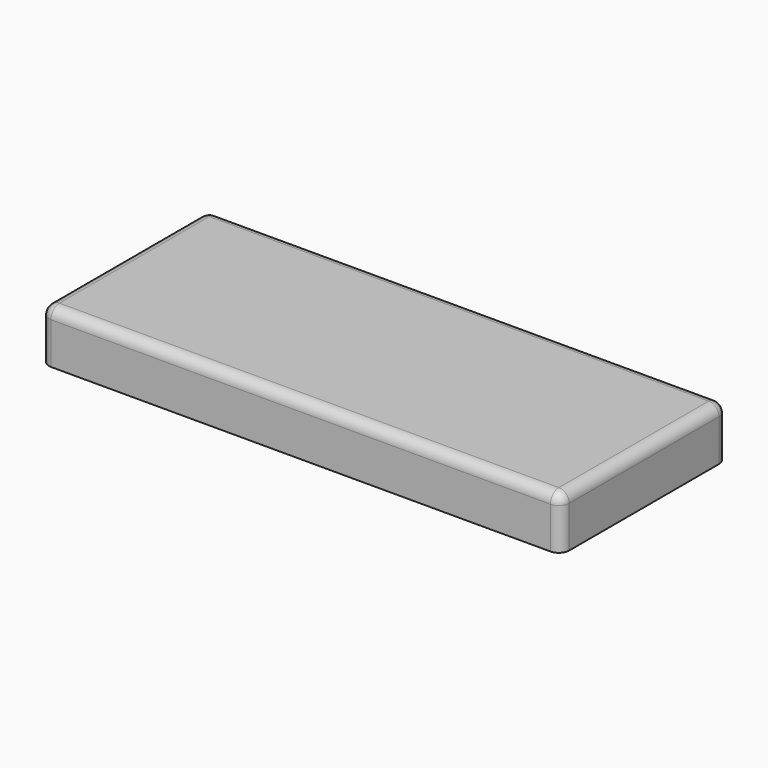
from build123d import *

# Parameters (mm, degrees)
F0_W        = 254
F0_H        = 101.6
F1_DEPTH    = 25.4
F2_R        = 5.08
F3_R        = 5.08
F4_T1_DEPTH = 33.02
F4_S5_W     = 5.08
F4_S5_H     = 5.08
F4_T6_DEPTH = 5.08
F5_T1_DEPTH = 33.02
F5_S5_W     = 5.08
F5_S5_H     = 5.08
F5_T6_DEPTH = 5.08


# Not quite as in the source:
# - a fillet or chamfer that OpenCascade refuses, or shapes differently, is made with other operations: its cross-section is extruded or revolved along the edge and cut away or added


with BuildPart() as f1:
    # F0 (on Top) → F1 (new body)
    with BuildSketch(Plane.XY):
        Rectangle(F0_W, F0_H)
    extrude(amount=F1_DEPTH)

    # F2
    f2_edges = [f1.edges().sort_by_distance(p)[0] for p in [
        (0, -50.8, 25.4),
    ]]
    fillet(f2_edges, radius=F2_R)

    # F3
    f3_edges = [f1.edges().sort_by_distance(p)[0] for p in [
        (127, 2.54, 25.4),
        (0, 50.8, 25.4),
        (-127, 2.54, 25.4),
    ]]
    fillet(f3_edges, radius=F3_R)

    # F4: fillet of radius 5.08 on 1 edges, made by hand

    # F4_s2 → F4_t1 (cut)
    with BuildSketch(Plane.XY.offset(-12.7)):
        with BuildLine():
            ThreePointArc((121.92, 50.8), (125.5121024484, 49.3121024484), (127, 45.72))
            Line((127, 45.72), (127, 50.8))
            Line((127, 50.8), (121.92, 50.8))
        make_face()
    extrude(amount=F4_T1_DEPTH, mode=Mode.SUBTRACT)


with BuildPart() as f4_tool4:
    # F4_s5 → F4_t6 (new body)
    with BuildSketch(Plane.XZ.offset(-45.72)):
        with Locations((124.46, 22.86)):
            Rectangle(F4_S5_W, F4_S5_H)
    extrude(amount=-F4_T6_DEPTH)

    # F4_s7 → F4_t8 (revolve, cut)
    with BuildSketch(Plane(origin=(121.92, 45.72, 20.32), x_dir=(-0.7071067812, 0, -0.7071067812), z_dir=(0.7071067812, 0, -0.7071067812))):
        with BuildLine():
            ThreePointArc((0, -5.08), (5.08, 0), (0, 5.08))
            Line((0, 5.08), (0, -5.08))
        make_face()
    revolve(axis=Axis((121.92, 45.72, 20.32), (0, 1, 0)), mode=Mode.SUBTRACT)


with BuildPart() as f1_1:
    add(f1.part)

    # F4_t3: cut F4_tool4
    add(f4_tool4.part, mode=Mode.SUBTRACT)

    # F5: fillet of radius 5.08 on 1 edges, made by hand

    # F5_s2 → F5_t1 (cut)
    with BuildSketch(Plane.XY.offset(-12.7)):
        with BuildLine():
            ThreePointArc((-127, 45.72), (-125.5121024484, 49.3121024484), (-121.92, 50.8))
            Line((-121.92, 50.8), (-127, 50.8))
            Line((-127, 50.8), (-127, 45.72))
        make_face()
    extrude(amount=F5_T1_DEPTH, mode=Mode.SUBTRACT)


with BuildPart() as f5_tool4:
    # F5_s5 → F5_t6 (new body)
    with BuildSketch(Plane.YZ.offset(-121.92)):
        with Locations((48.26, 22.86)):
            Rectangle(F5_S5_W, F5_S5_H)
    extrude(amount=-F5_T6_DEPTH)

    # F5_s7 → F5_t8 (revolve, cut)
    with BuildSketch(Plane(origin=(-121.92, 45.72, 20.32), x_dir=(0, -0.7071067812, -0.7071067812), z_dir=(0, 0.7071067812, -0.7071067812))):
        with BuildLine():
            ThreePointArc((0, -5.08), (5.08, 0), (0, 5.08))
            Line((0, 5.08), (0, -5.08))
        make_face()
    revolve(axis=Axis((-121.92, 45.72, 20.32), (-1, 0, 0)), mode=Mode.SUBTRACT)


with BuildPart() as f1_2:
    add(f1_1.part)

    # F5_t3: cut F5_tool4
    add(f5_tool4.part, mode=Mode.SUBTRACT)


solid = f1_2.part
